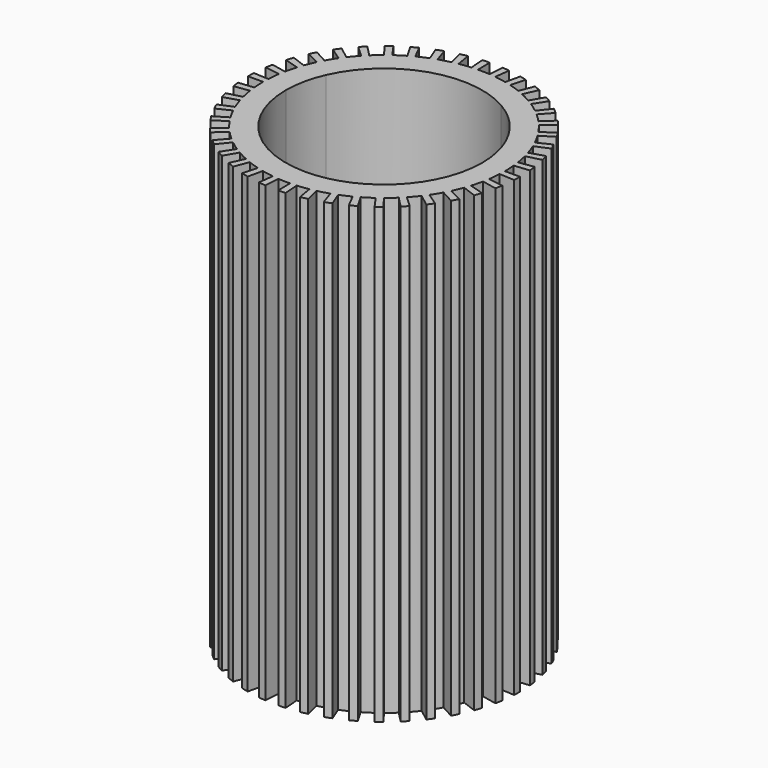
from build123d import *
from build123d import SkipClean  # not in build123d's __all__

# Parameters (mm, degrees)
F1_DEPTH = 1.5
F2_DEPTH = 30
F3_DEPTH = 10
F4_DEPTH = 10
F5_DEPTH = 1.5


with BuildPart() as f1:
    # F0 (on Top) → F1 (new body)
    with BuildSketch(Plane.XY):
        with BuildLine():
            ThreePointArc((-6.5, 0), (-4.3493489413, -4.8304413656), (0.6794350112, -6.4643923199))
            Line((0.6794350112, -6.4643923199), (0.3135853898, -2.9835656861))
            ThreePointArc((0.3135853898, -2.9835656861), (-2.0073918191, -2.2294344764), (-3, 0))
            Line((-3, 0), (-6.5, 0))
        make_face()
        with BuildLine():
            Line((-2.7406363729, 1.2202099292), (-5.9380454747, 2.64378818))
            ThreePointArc((-5.9380454747, 2.64378818), (-6.3579594048, 1.3514259903), (-6.5, 0))
            Line((-6.5, 0), (-3, 0))
            ThreePointArc((-3, 0), (-2.9344428022, 0.6237350725), (-2.7406363729, 1.2202099292))
        make_face()
        with BuildLine():
            Line((1.5, 2.5980762114), (3.25, 5.6291651246))
            ThreePointArc((3.25, 5.6291651246), (-2.0086104634, 6.1818673559), (-5.9380454747, 2.64378818))
            Line((-5.9380454747, 2.64378818), (-2.7406363729, 1.2202099292))
            ThreePointArc((-2.7406363729, 1.2202099292), (-0.9270509831, 2.8531695489), (1.5, 2.5980762114))
        make_face()
        with BuildLine():
            Line((2.4270509831, 1.7633557569), (5.2586104634, 3.8206041399))
            ThreePointArc((5.2586104634, 3.8206041399), (4.3493489413, 4.8304413656), (3.25, 5.6291651246))
            Line((3.25, 5.6291651246), (1.5, 2.5980762114))
            ThreePointArc((1.5, 2.5980762114), (2.0073918191, 2.2294344764), (2.4270509831, 1.7633557569))
        make_face()
        with BuildLine():
            ThreePointArc((3.25, -5.6291651246), (5.6291651246, -3.25), (6.5, 0))
            ThreePointArc((6.5, 0), (6.1818673559, 2.0086104634), (5.2586104634, 3.8206041399))
            Line((5.2586104634, 3.8206041399), (2.4270509831, 1.7633557569))
            ThreePointArc((2.4270509831, 1.7633557569), (2.8531695489, 0.9270509831), (3, 0))
            ThreePointArc((3, 0), (2.5980762114, -1.5), (1.5, -2.5980762114))
            Line((1.5, -2.5980762114), (3.25, -5.6291651246))
        make_face()
        with BuildLine():
            ThreePointArc((0.6794350112, -6.4643923199), (2.0086104634, -6.1818673559), (3.25, -5.6291651246))
            Line((3.25, -5.6291651246), (1.5, -2.5980762114))
            ThreePointArc((1.5, -2.5980762114), (0.9270509831, -2.8531695489), (0.3135853898, -2.9835656861))
            Line((0.3135853898, -2.9835656861), (0.6794350112, -6.4643923199))
        make_face()
    extrude(amount=F1_DEPTH)

    # F0 (on Top) → F2 (join)
    with BuildSketch(Plane.XY):
        with BuildLine():
            ThreePointArc((7.989036278, -0.4186876499), (7.9972585998, -0.2094155865), (8, 0))
            ThreePointArc((8, 0), (7.9905462891, 0.3888058656), (7.9622074997, 0.7766928166))
            ThreePointArc((7.9622074997, 0.7766928166), (7.9391476024, 0.9848529575), (7.9106466098, 1.1923381294))
            ThreePointArc((7.9106466098, 1.1923381294), (7.8433499818, 1.5753923522), (7.757516163, 1.9547232491))
            ThreePointArc((7.757516163, 1.9547232491), (7.7036891665, 2.1571215139), (7.6445824463, 2.3580413953))
            ThreePointArc((7.6445824463, 2.3580413953), (7.5209461966, 2.726787177), (7.3795347341, 3.0890883943))
            ThreePointArc((7.3795347341, 3.0890883943), (7.2961430447, 3.2812035401), (7.2077509432, 3.4710699129))
            ThreePointArc((7.2077509432, 3.4710699129), (7.0305369013, 3.8172700821), (6.8367066936, 4.1544484093))
            ThreePointArc((6.8367066936, 4.1544484093), (6.7256131437, 4.3319889013), (6.6099101945, 4.5065604645))
            ThreePointArc((6.6099101945, 4.5065604645), (6.3830770293, 4.8224814814), (6.1411579229, 5.1270049119))
            ThreePointArc((6.1411579229, 5.1270049119), (6.0048441589, 5.2860047888), (5.8644149746, 5.4413819022))
            ThreePointArc((5.8644149746, 5.4413819022), (5.5930297641, 5.7199666133), (5.3084258321, 5.9850325968))
            ThreePointArc((5.3084258321, 5.9850325968), (5.1499368782, 6.1219400643), (4.9879184149, 6.2546518597))
            ThreePointArc((4.9879184149, 6.2546518597), (4.6780434563, 6.4896771431), (4.3571122801, 6.7093645436))
            ThreePointArc((4.3571122801, 6.7093645436), (4.1799885177, 6.8211213148), (4, 6.9282032303))
            ThreePointArc((4, 6.9282032303), (3.6585573878, 7.1144190093), (3.3084680397, 7.2838203733))
            ThreePointArc((3.3084680397, 7.2838203733), (3.116666121, 7.3679299868), (2.9227281949, 7.4469899892))
            ThreePointArc((2.9227281949, 7.4469899892), (2.5573451929, 7.5802365111), (2.1859180904, 7.695567692))
            ThreePointArc((2.1859180904, 7.695567692), (1.9837225532, 7.750151278), (1.7801674717, 7.7994232975))
            ThreePointArc((1.7801674717, 7.7994232975), (1.3990061323, 7.8767240552), (1.0145383431, 7.935408745))
            ThreePointArc((1.0145383431, 7.935408745), (0.8064659016, 7.9592469964), (0.5978407487, 7.9776303774))
            ThreePointArc((0.5978407487, 7.9776303774), (0.2094155865, 7.9972585998), (-0.1795045144, 7.9979858795))
            ThreePointArc((-0.1795045144, 7.9979858795), (-0.3888058656, 7.9905462891), (-0.5978407487, 7.9776303774))
            ThreePointArc((-0.5978407487, 7.9776303774), (-0.9848529575, 7.9391476024), (-1.3695375376, 7.8819012258))
            ThreePointArc((-1.3695375376, 7.8819012258), (-1.5753923522, 7.8433499818), (-1.7801674717, 7.7994232975))
            ThreePointArc((-1.7801674717, 7.7994232975), (-2.1571215139, 7.7036891665), (-2.5289773553, 7.5897479231))
            ThreePointArc((-2.5289773553, 7.5897479231), (-2.726787177, 7.5209461966), (-2.9227281949, 7.4469899892))
            ThreePointArc((-2.9227281949, 7.4469899892), (-3.2812035401, 7.2961430447), (-3.6319239979, 7.1280521935))
            ThreePointArc((-3.6319239979, 7.1280521935), (-3.8172700821, 7.0305369013), (-4, 6.9282032303))
            ThreePointArc((-4, 6.9282032303), (-4.3319889013, 6.7256131437), (-4.65373946, 6.5071275567))
            ThreePointArc((-4.65373946, 6.5071275567), (-4.8224814814, 6.3830770293), (-4.9879184149, 6.2546518597))
            ThreePointArc((-4.9879184149, 6.2546518597), (-5.2860047888, 6.0048441589), (-5.5715980726, 5.7408444429))
            ThreePointArc((-5.5715980726, 5.7408444429), (-5.7199666133, 5.5930297641), (-5.8644149746, 5.4413819022))
            ThreePointArc((-5.8644149746, 5.4413819022), (-6.1219400643, 5.1499368782), (-6.3649963911, 4.8463203507))
            ThreePointArc((-6.3649963911, 4.8463203507), (-6.4896771431, 4.6780434563), (-6.6099101945, 4.5065604645))
            ThreePointArc((-6.6099101945, 4.5065604645), (-6.8211213148, 4.1799885177), (-7.016211208, 3.8435374702))
            ThreePointArc((-7.016211208, 3.8435374702), (-7.1144190093, 3.6585573878), (-7.2077509432, 3.4710699129))
            ThreePointArc((-7.2077509432, 3.4710699129), (-7.3679299868, 3.116666121), (-7.5106954604, 2.7548963139))
            ThreePointArc((-7.5106954604, 2.7548963139), (-7.5802365111, 2.5573451929), (-7.6445824463, 2.3580413953))
            ThreePointArc((-7.6445824463, 2.3580413953), (-7.750151278, 1.9837225532), (-7.8374031874, 1.6047153263))
            ThreePointArc((-7.8374031874, 1.6047153263), (-7.8767240552, 1.3990061323), (-7.9106466098, 1.1923381294))
            ThreePointArc((-7.9106466098, 1.1923381294), (-7.9592469964, 0.8064659016), (-7.989036278, 0.4186876499))
            ThreePointArc((-7.989036278, 0.4186876499), (-7.9972585998, 0.2094155865), (-8, 0))
            ThreePointArc((-8, 0), (-7.9905462891, -0.3888058656), (-7.9622074997, -0.7766928166))
            ThreePointArc((-7.9622074997, -0.7766928166), (-7.9391476024, -0.9848529575), (-7.9106466098, -1.1923381294))
            ThreePointArc((-7.9106466098, -1.1923381294), (-7.8433499818, -1.5753923522), (-7.757516163, -1.9547232491))
            ThreePointArc((-7.757516163, -1.9547232491), (-7.7036891665, -2.1571215139), (-7.6445824463, -2.3580413953))
            ThreePointArc((-7.6445824463, -2.3580413953), (-7.5209461966, -2.726787177), (-7.3795347341, -3.0890883943))
            ThreePointArc((-7.3795347341, -3.0890883943), (-7.2961430447, -3.2812035401), (-7.2077509432, -3.4710699129))
            ThreePointArc((-7.2077509432, -3.4710699129), (-7.0305369013, -3.8172700821), (-6.8367066936, -4.1544484093))
            ThreePointArc((-6.8367066936, -4.1544484093), (-6.7256131437, -4.3319889013), (-6.6099101945, -4.5065604645))
            ThreePointArc((-6.6099101945, -4.5065604645), (-6.3830770293, -4.8224814814), (-6.1411579229, -5.1270049119))
            ThreePointArc((-6.1411579229, -5.1270049119), (-6.0048441589, -5.2860047888), (-5.8644149746, -5.4413819022))
            ThreePointArc((-5.8644149746, -5.4413819022), (-5.5930297641, -5.7199666133), (-5.3084258321, -5.9850325968))
            ThreePointArc((-5.3084258321, -5.9850325968), (-5.1499368782, -6.1219400643), (-4.9879184149, -6.2546518597))
            ThreePointArc((-4.9879184149, -6.2546518597), (-4.6780434563, -6.4896771431), (-4.3571122801, -6.7093645436))
            ThreePointArc((-4.3571122801, -6.7093645436), (-4.1799885177, -6.8211213148), (-4, -6.9282032303))
            ThreePointArc((-4, -6.9282032303), (-3.6585573878, -7.1144190093), (-3.3084680397, -7.2838203733))
            ThreePointArc((-3.3084680397, -7.2838203733), (-3.116666121, -7.3679299868), (-2.9227281949, -7.4469899892))
            ThreePointArc((-2.9227281949, -7.4469899892), (-2.5573451929, -7.5802365111), (-2.1859180904, -7.695567692))
            ThreePointArc((-2.1859180904, -7.695567692), (-1.9837225532, -7.750151278), (-1.7801674717, -7.7994232975))
            ThreePointArc((-1.7801674717, -7.7994232975), (-1.3990061323, -7.8767240552), (-1.0145383431, -7.935408745))
            ThreePointArc((-1.0145383431, -7.935408745), (-0.8064659016, -7.9592469964), (-0.5978407487, -7.9776303774))
            ThreePointArc((-0.5978407487, -7.9776303774), (-0.2094155865, -7.9972585998), (0.1795045144, -7.9979858795))
            ThreePointArc((0.1795045144, -7.9979858795), (0.3888058656, -7.9905462891), (0.5978407487, -7.9776303774))
            ThreePointArc((0.5978407487, -7.9776303774), (0.9848529575, -7.9391476024), (1.3695375376, -7.8819012258))
            ThreePointArc((1.3695375376, -7.8819012258), (1.5753923522, -7.8433499818), (1.7801674717, -7.7994232975))
            ThreePointArc((1.7801674717, -7.7994232975), (2.1571215139, -7.7036891665), (2.5289773553, -7.5897479231))
            ThreePointArc((2.5289773553, -7.5897479231), (2.726787177, -7.5209461966), (2.9227281949, -7.4469899892))
            ThreePointArc((2.9227281949, -7.4469899892), (3.2812035401, -7.2961430447), (3.6319239979, -7.1280521935))
            ThreePointArc((3.6319239979, -7.1280521935), (3.8172700821, -7.0305369013), (4, -6.9282032303))
            ThreePointArc((4, -6.9282032303), (4.3319889013, -6.7256131437), (4.65373946, -6.5071275567))
            ThreePointArc((4.65373946, -6.5071275567), (4.8224814814, -6.3830770293), (4.9879184149, -6.2546518597))
            ThreePointArc((4.9879184149, -6.2546518597), (5.2860047888, -6.0048441589), (5.5715980726, -5.7408444429))
            ThreePointArc((5.5715980726, -5.7408444429), (5.7199666133, -5.5930297641), (5.8644149746, -5.4413819022))
            ThreePointArc((5.8644149746, -5.4413819022), (6.1219400643, -5.1499368782), (6.3649963911, -4.8463203507))
            ThreePointArc((6.3649963911, -4.8463203507), (6.4896771431, -4.6780434563), (6.6099101945, -4.5065604645))
            ThreePointArc((6.6099101945, -4.5065604645), (6.8211213148, -4.1799885177), (7.016211208, -3.8435374702))
            ThreePointArc((7.016211208, -3.8435374702), (7.1144190093, -3.6585573878), (7.2077509432, -3.4710699129))
            ThreePointArc((7.2077509432, -3.4710699129), (7.3679299868, -3.116666121), (7.5106954604, -2.7548963139))
            ThreePointArc((7.5106954604, -2.7548963139), (7.5802365111, -2.5573451929), (7.6445824463, -2.3580413953))
            ThreePointArc((7.6445824463, -2.3580413953), (7.750151278, -1.9837225532), (7.8374031874, -1.6047153263))
            ThreePointArc((7.8374031874, -1.6047153263), (7.8767240552, -1.3990061323), (7.9106466098, -1.1923381294))
            ThreePointArc((7.9106466098, -1.1923381294), (7.9592469964, -0.8064659016), (7.989036278, -0.4186876499))
        make_face()
        with BuildLine():
            ThreePointArc((5.2586104634, 3.8206041399), (6.1818673559, 2.0086104634), (6.5, 0))
            ThreePointArc((6.5, 0), (5.6291651246, -3.25), (3.25, -5.6291651246))
            ThreePointArc((3.25, -5.6291651246), (2.0086104634, -6.1818673559), (0.6794350112, -6.4643923199))
            ThreePointArc((0.6794350112, -6.4643923199), (-4.3493489413, -4.8304413656), (-6.5, 0))
            ThreePointArc((-6.5, 0), (-6.3579594048, 1.3514259903), (-5.9380454747, 2.64378818))
            ThreePointArc((-5.9380454747, 2.64378818), (-2.0086104634, 6.1818673559), (3.25, 5.6291651246))
            ThreePointArc((3.25, 5.6291651246), (4.3493489413, 4.8304413656), (5.2586104634, 3.8206041399))
        make_face(mode=Mode.SUBTRACT)
        with BuildLine():
            ThreePointArc((-6.6099101945, 4.5065604645), (-6.4896771431, 4.6780434563), (-6.3649963911, 4.8463203507))
            Line((-6.3649963911, 4.8463203507), (-7.1606209399, 5.4521103946))
            ThreePointArc((-7.1606209399, 5.4521103946), (-7.3008867859, 5.2627988883), (-7.4361489688, 5.0698805226))
            Line((-7.4361489688, 5.0698805226), (-6.6099101945, 4.5065604645))
        make_face()
        with BuildLine():
            ThreePointArc((-5.8644149746, 5.4413819022), (-5.7199666133, 5.5930297641), (-5.5715980726, 5.7408444429))
            Line((-5.5715980726, 5.7408444429), (-6.2680478317, 6.4584499982))
            ThreePointArc((-6.2680478317, 6.4584499982), (-6.43496244, 6.2921584847), (-6.5974668465, 6.1215546399))
            Line((-6.5974668465, 6.1215546399), (-5.8644149746, 5.4413819022))
        make_face()
        with BuildLine():
            ThreePointArc((-4.9879184149, 6.2546518597), (-4.8224814814, 6.3830770293), (-4.65373946, 6.5071275567))
            Line((-4.65373946, 6.5071275567), (-5.2354568925, 7.3205185012))
            ThreePointArc((-5.2354568925, 7.3205185012), (-5.4252916666, 7.1809616579), (-5.6114082167, 7.0364833422))
            Line((-5.6114082167, 7.0364833422), (-4.9879184149, 6.2546518597))
        make_face()
        with BuildLine():
            ThreePointArc((-4, 6.9282032303), (-3.8172700821, 7.0305369013), (-3.6319239979, 7.1280521935))
            Line((-3.6319239979, 7.1280521935), (-4.0859144977, 8.0190587177))
            ThreePointArc((-4.0859144977, 8.0190587177), (-4.2944288423, 7.909354014), (-4.5, 7.7942286341))
            Line((-4.5, 7.7942286341), (-4, 6.9282032303))
        make_face()
        with BuildLine():
            ThreePointArc((-2.9227281949, 7.4469899892), (-2.726787177, 7.5209461966), (-2.5289773553, 7.5897479231))
            Line((-2.5289773553, 7.5897479231), (-2.8450995247, 8.5384664135))
            ThreePointArc((-2.8450995247, 8.5384664135), (-3.0676355741, 8.4610644711), (-3.2880692193, 8.3778637378))
            Line((-3.2880692193, 8.3778637378), (-2.9227281949, 7.4469899892))
        make_face()
        with BuildLine():
            ThreePointArc((-1.7801674717, 7.7994232975), (-1.5753923522, 7.8433499818), (-1.3695375376, 7.8819012258))
            Line((-1.3695375376, 7.8819012258), (-1.5407297298, 8.867138879))
            ThreePointArc((-1.5407297298, 8.867138879), (-1.7723163963, 8.8237687295), (-2.0026884056, 8.7743512096))
            Line((-2.0026884056, 8.7743512096), (-1.7801674717, 7.7994232975))
        make_face()
        with BuildLine():
            ThreePointArc((-0.5978407487, 7.9776303774), (-0.3888058656, 7.9905462891), (-0.1795045144, 7.9979858795))
            Line((-0.1795045144, 7.9979858795), (-0.2019425787, 8.9977341145))
            ThreePointArc((-0.2019425787, 8.9977341145), (-0.4374065988, 8.9893645753), (-0.6725708423, 8.9748341746))
            Line((-0.6725708423, 8.9748341746), (-0.5978407487, 7.9776303774))
        make_face()
        with BuildLine():
            ThreePointArc((0.5978407487, 7.9776303774), (0.8064659016, 7.9592469964), (1.0145383431, 7.935408745))
            Line((1.0145383431, 7.935408745), (1.141355636, 8.9273348381))
            ThreePointArc((1.141355636, 8.9273348381), (0.9072741393, 8.9541528709), (0.6725708423, 8.9748341746))
            Line((0.6725708423, 8.9748341746), (0.5978407487, 7.9776303774))
        make_face()
        with BuildLine():
            ThreePointArc((1.7801674717, 7.7994232975), (1.9837225532, 7.750151278), (2.1859180904, 7.695567692))
            Line((2.1859180904, 7.695567692), (2.4591578517, 8.6575136535))
            ThreePointArc((2.4591578517, 8.6575136535), (2.2316878724, 8.7189201878), (2.0026884056, 8.7743512096))
            Line((2.0026884056, 8.7743512096), (1.7801674717, 7.7994232975))
        make_face()
        with BuildLine():
            ThreePointArc((2.9227281949, 7.4469899892), (3.116666121, 7.3679299868), (3.3084680397, 7.2838203733))
            Line((3.3084680397, 7.2838203733), (3.7220265447, 8.1942979199))
            ThreePointArc((3.7220265447, 8.1942979199), (3.5062493861, 8.2889212352), (3.2880692193, 8.3778637378))
            Line((3.2880692193, 8.3778637378), (2.9227281949, 7.4469899892))
        make_face()
        with BuildLine():
            ThreePointArc((4, 6.9282032303), (4.1799885177, 6.8211213148), (4.3571122801, 6.7093645436))
            Line((4.3571122801, 6.7093645436), (4.9017513151, 7.5480351115))
            ThreePointArc((4.9017513151, 7.5480351115), (4.7024870824, 7.6737614792), (4.5, 7.7942286341))
            Line((4.5, 7.7942286341), (4, 6.9282032303))
        make_face()
        with BuildLine():
            ThreePointArc((4.9879184149, 6.2546518597), (5.1499368782, 6.1219400643), (5.3084258321, 5.9850325968))
            Line((5.3084258321, 5.9850325968), (5.9719790611, 6.7331616714))
            ThreePointArc((5.9719790611, 6.7331616714), (5.793678988, 6.8871825723), (5.6114082167, 7.0364833422))
            Line((5.6114082167, 7.0364833422), (4.9879184149, 6.2546518597))
        make_face()
        with BuildLine():
            ThreePointArc((5.8644149746, 5.4413819022), (6.0048441589, 5.2860047888), (6.1411579229, 5.1270049119))
            Line((6.1411579229, 5.1270049119), (6.9088026632, 5.7678805259))
            ThreePointArc((6.9088026632, 5.7678805259), (6.7554496787, 5.9467553874), (6.5974668465, 6.1215546399))
            Line((6.5974668465, 6.1215546399), (5.8644149746, 5.4413819022))
        make_face()
        with BuildLine():
            ThreePointArc((6.6099101945, 4.5065604645), (6.7256131437, 4.3319889013), (6.8367066936, 4.1544484093))
            Line((6.8367066936, 4.1544484093), (7.6912950303, 4.6737544605))
            ThreePointArc((7.6912950303, 4.6737544605), (7.5663147867, 4.873487514), (7.4361489688, 5.0698805226))
            Line((7.4361489688, 5.0698805226), (6.6099101945, 4.5065604645))
        make_face()
        with BuildLine():
            ThreePointArc((7.2077509432, 3.4710699129), (7.2961430447, 3.2812035401), (7.3795347341, 3.0890883943))
            Line((7.3795347341, 3.0890883943), (8.3019765759, 3.4752244436))
            ThreePointArc((8.3019765759, 3.4752244436), (8.2081609253, 3.6913539826), (8.1087198111, 3.9049536521))
            Line((8.1087198111, 3.9049536521), (7.2077509432, 3.4710699129))
        make_face()
        with BuildLine():
            ThreePointArc((7.6445824463, 2.3580413953), (7.7036891665, 2.1571215139), (7.757516163, 1.9547232491))
            Line((7.757516163, 1.9547232491), (8.7272056834, 2.1990636552))
            ThreePointArc((8.7272056834, 2.1990636552), (8.6666503123, 2.4267617031), (8.6001552521, 2.6527965697))
            Line((8.6001552521, 2.6527965697), (7.6445824463, 2.3580413953))
        make_face()
        with BuildLine():
            ThreePointArc((7.9106466098, 1.1923381294), (7.9391476024, 0.9848529575), (7.9622074997, 0.7766928166))
            Line((7.9622074997, 0.7766928166), (8.9574834372, 0.8737794187))
            ThreePointArc((8.9574834372, 0.8737794187), (8.9315410527, 1.1079595772), (8.899477436, 1.3413803956))
            Line((8.899477436, 1.3413803956), (7.9106466098, 1.1923381294))
        make_face()
        with BuildLine():
            Line((9, 0), (8, 0))
            ThreePointArc((8, 0), (7.9972585998, -0.2094155865), (7.989036278, -0.4186876499))
            Line((7.989036278, -0.4186876499), (8.9876658128, -0.4710236062))
            ThreePointArc((8.9876658128, -0.4710236062), (8.9969159248, -0.2355925348), (9, 0))
        make_face()
        with BuildLine():
            Line((8.899477436, -1.3413803956), (7.9106466098, -1.1923381294))
            ThreePointArc((7.9106466098, -1.1923381294), (7.8767240552, -1.3990061323), (7.8374031874, -1.6047153263))
            Line((7.8374031874, -1.6047153263), (8.8170785858, -1.805304742))
            ThreePointArc((8.8170785858, -1.805304742), (8.8613145621, -1.5738818988), (8.899477436, -1.3413803956))
        make_face()
        with BuildLine():
            Line((8.6001552521, -2.6527965697), (7.6445824463, -2.3580413953))
            ThreePointArc((7.6445824463, -2.3580413953), (7.5802365111, -2.5573451929), (7.5106954604, -2.7548963139))
            Line((7.5106954604, -2.7548963139), (8.449532393, -3.0992583532))
            ThreePointArc((8.449532393, -3.0992583532), (8.527766075, -2.877013342), (8.6001552521, -2.6527965697))
        make_face()
        with BuildLine():
            Line((8.1087198111, -3.9049536521), (7.2077509432, -3.4710699129))
            ThreePointArc((7.2077509432, -3.4710699129), (7.1144190093, -3.6585573878), (7.016211208, -3.8435374702))
            Line((7.016211208, -3.8435374702), (7.893237609, -4.323979654))
            ThreePointArc((7.893237609, -4.323979654), (8.0037213855, -4.1158770613), (8.1087198111, -3.9049536521))
        make_face()
        with BuildLine():
            Line((7.4361489688, -5.0698805226), (6.6099101945, -4.5065604645))
            ThreePointArc((6.6099101945, -4.5065604645), (6.4896771431, -4.6780434563), (6.3649963911, -4.8463203507))
            Line((6.3649963911, -4.8463203507), (7.1606209399, -5.4521103946))
            ThreePointArc((7.1606209399, -5.4521103946), (7.3008867859, -5.2627988883), (7.4361489688, -5.0698805226))
        make_face()
        with BuildLine():
            Line((6.5974668465, -6.1215546399), (5.8644149746, -5.4413819022))
            ThreePointArc((5.8644149746, -5.4413819022), (5.7199666133, -5.5930297641), (5.5715980726, -5.7408444429))
            Line((5.5715980726, -5.7408444429), (6.2680478317, -6.4584499982))
            ThreePointArc((6.2680478317, -6.4584499982), (6.43496244, -6.2921584847), (6.5974668465, -6.1215546399))
        make_face()
        with BuildLine():
            Line((5.6114082167, -7.0364833422), (4.9879184149, -6.2546518597))
            ThreePointArc((4.9879184149, -6.2546518597), (4.8224814814, -6.3830770293), (4.65373946, -6.5071275567))
            Line((4.65373946, -6.5071275567), (5.2354568925, -7.3205185012))
            ThreePointArc((5.2354568925, -7.3205185012), (5.4252916666, -7.1809616579), (5.6114082167, -7.0364833422))
        make_face()
        with BuildLine():
            Line((4.5, -7.7942286341), (4, -6.9282032303))
            ThreePointArc((4, -6.9282032303), (3.8172700821, -7.0305369013), (3.6319239979, -7.1280521935))
            Line((3.6319239979, -7.1280521935), (4.0859144977, -8.0190587177))
            ThreePointArc((4.0859144977, -8.0190587177), (4.2944288423, -7.909354014), (4.5, -7.7942286341))
        make_face()
        with BuildLine():
            Line((3.2880692193, -8.3778637378), (2.9227281949, -7.4469899892))
            ThreePointArc((2.9227281949, -7.4469899892), (2.726787177, -7.5209461966), (2.5289773553, -7.5897479231))
            Line((2.5289773553, -7.5897479231), (2.8450995247, -8.5384664135))
            ThreePointArc((2.8450995247, -8.5384664135), (3.0676355741, -8.4610644711), (3.2880692193, -8.3778637378))
        make_face()
        with BuildLine():
            Line((2.0026884056, -8.7743512096), (1.7801674717, -7.7994232975))
            ThreePointArc((1.7801674717, -7.7994232975), (1.5753923522, -7.8433499818), (1.3695375376, -7.8819012258))
            Line((1.3695375376, -7.8819012258), (1.5407297298, -8.867138879))
            ThreePointArc((1.5407297298, -8.867138879), (1.7723163963, -8.8237687295), (2.0026884056, -8.7743512096))
        make_face()
        with BuildLine():
            Line((0.6725708423, -8.9748341746), (0.5978407487, -7.9776303774))
            ThreePointArc((0.5978407487, -7.9776303774), (0.3888058656, -7.9905462891), (0.1795045144, -7.9979858795))
            Line((0.1795045144, -7.9979858795), (0.2019425787, -8.9977341145))
            ThreePointArc((0.2019425787, -8.9977341145), (0.4374065988, -8.9893645753), (0.6725708423, -8.9748341746))
        make_face()
        with BuildLine():
            Line((-0.6725708423, -8.9748341746), (-0.5978407487, -7.9776303774))
            ThreePointArc((-0.5978407487, -7.9776303774), (-0.8064659016, -7.9592469964), (-1.0145383431, -7.935408745))
            Line((-1.0145383431, -7.935408745), (-1.141355636, -8.9273348381))
            ThreePointArc((-1.141355636, -8.9273348381), (-0.9072741393, -8.9541528709), (-0.6725708423, -8.9748341746))
        make_face()
        with BuildLine():
            Line((-2.0026884056, -8.7743512096), (-1.7801674717, -7.7994232975))
            ThreePointArc((-1.7801674717, -7.7994232975), (-1.9837225532, -7.750151278), (-2.1859180904, -7.695567692))
            Line((-2.1859180904, -7.695567692), (-2.4591578517, -8.6575136535))
            ThreePointArc((-2.4591578517, -8.6575136535), (-2.2316878724, -8.7189201878), (-2.0026884056, -8.7743512096))
        make_face()
        with BuildLine():
            Line((-3.2880692193, -8.3778637378), (-2.9227281949, -7.4469899892))
            ThreePointArc((-2.9227281949, -7.4469899892), (-3.116666121, -7.3679299868), (-3.3084680397, -7.2838203733))
            Line((-3.3084680397, -7.2838203733), (-3.7220265447, -8.1942979199))
            ThreePointArc((-3.7220265447, -8.1942979199), (-3.5062493861, -8.2889212352), (-3.2880692193, -8.3778637378))
        make_face()
        with BuildLine():
            Line((-4.5, -7.7942286341), (-4, -6.9282032303))
            ThreePointArc((-4, -6.9282032303), (-4.1799885177, -6.8211213148), (-4.3571122801, -6.7093645436))
            Line((-4.3571122801, -6.7093645436), (-4.9017513151, -7.5480351115))
            ThreePointArc((-4.9017513151, -7.5480351115), (-4.7024870824, -7.6737614792), (-4.5, -7.7942286341))
        make_face()
        with BuildLine():
            Line((-5.6114082167, -7.0364833422), (-4.9879184149, -6.2546518597))
            ThreePointArc((-4.9879184149, -6.2546518597), (-5.1499368782, -6.1219400643), (-5.3084258321, -5.9850325968))
            Line((-5.3084258321, -5.9850325968), (-5.9719790611, -6.7331616714))
            ThreePointArc((-5.9719790611, -6.7331616714), (-5.793678988, -6.8871825723), (-5.6114082167, -7.0364833422))
        make_face()
        with BuildLine():
            Line((-6.5974668465, -6.1215546399), (-5.8644149746, -5.4413819022))
            ThreePointArc((-5.8644149746, -5.4413819022), (-6.0048441589, -5.2860047888), (-6.1411579229, -5.1270049119))
            Line((-6.1411579229, -5.1270049119), (-6.9088026632, -5.7678805259))
            ThreePointArc((-6.9088026632, -5.7678805259), (-6.7554496787, -5.9467553874), (-6.5974668465, -6.1215546399))
        make_face()
        with BuildLine():
            Line((-7.4361489688, -5.0698805226), (-6.6099101945, -4.5065604645))
            ThreePointArc((-6.6099101945, -4.5065604645), (-6.7256131437, -4.3319889013), (-6.8367066936, -4.1544484093))
            Line((-6.8367066936, -4.1544484093), (-7.6912950303, -4.6737544605))
            ThreePointArc((-7.6912950303, -4.6737544605), (-7.5663147867, -4.873487514), (-7.4361489688, -5.0698805226))
        make_face()
        with BuildLine():
            Line((-8.1087198111, -3.9049536521), (-7.2077509432, -3.4710699129))
            ThreePointArc((-7.2077509432, -3.4710699129), (-7.2961430447, -3.2812035401), (-7.3795347341, -3.0890883943))
            Line((-7.3795347341, -3.0890883943), (-8.3019765759, -3.4752244436))
            ThreePointArc((-8.3019765759, -3.4752244436), (-8.2081609253, -3.6913539826), (-8.1087198111, -3.9049536521))
        make_face()
        with BuildLine():
            Line((-8.6001552521, -2.6527965697), (-7.6445824463, -2.3580413953))
            ThreePointArc((-7.6445824463, -2.3580413953), (-7.7036891665, -2.1571215139), (-7.757516163, -1.9547232491))
            Line((-7.757516163, -1.9547232491), (-8.7272056834, -2.1990636552))
            ThreePointArc((-8.7272056834, -2.1990636552), (-8.6666503123, -2.4267617031), (-8.6001552521, -2.6527965697))
        make_face()
        with BuildLine():
            Line((-8.899477436, -1.3413803956), (-7.9106466098, -1.1923381294))
            ThreePointArc((-7.9106466098, -1.1923381294), (-7.9391476024, -0.9848529575), (-7.9622074997, -0.7766928166))
            Line((-7.9622074997, -0.7766928166), (-8.9574834372, -0.8737794187))
            ThreePointArc((-8.9574834372, -0.8737794187), (-8.9315410527, -1.1079595772), (-8.899477436, -1.3413803956))
        make_face()
        with BuildLine():
            ThreePointArc((-8, 0), (-7.9972585998, 0.2094155865), (-7.989036278, 0.4186876499))
            Line((-7.989036278, 0.4186876499), (-8.9876658128, 0.4710236062))
            ThreePointArc((-8.9876658128, 0.4710236062), (-8.9969159248, 0.2355925348), (-9, 0))
            Line((-9, 0), (-8, 0))
        make_face()
        with BuildLine():
            ThreePointArc((-7.9106466098, 1.1923381294), (-7.8767240552, 1.3990061323), (-7.8374031874, 1.6047153263))
            Line((-7.8374031874, 1.6047153263), (-8.8170785858, 1.805304742))
            ThreePointArc((-8.8170785858, 1.805304742), (-8.8613145621, 1.5738818988), (-8.899477436, 1.3413803956))
            Line((-8.899477436, 1.3413803956), (-7.9106466098, 1.1923381294))
        make_face()
        with BuildLine():
            ThreePointArc((-7.6445824463, 2.3580413953), (-7.5802365111, 2.5573451929), (-7.5106954604, 2.7548963139))
            Line((-7.5106954604, 2.7548963139), (-8.449532393, 3.0992583532))
            ThreePointArc((-8.449532393, 3.0992583532), (-8.527766075, 2.877013342), (-8.6001552521, 2.6527965697))
            Line((-8.6001552521, 2.6527965697), (-7.6445824463, 2.3580413953))
        make_face()
        with BuildLine():
            ThreePointArc((-7.2077509432, 3.4710699129), (-7.1144190093, 3.6585573878), (-7.016211208, 3.8435374702))
            Line((-7.016211208, 3.8435374702), (-7.893237609, 4.323979654))
            ThreePointArc((-7.893237609, 4.323979654), (-8.0037213855, 4.1158770613), (-8.1087198111, 3.9049536521))
            Line((-8.1087198111, 3.9049536521), (-7.2077509432, 3.4710699129))
        make_face()
    extrude(amount=F2_DEPTH)

    # F0 (on Top) → F3 (join)
    with BuildSketch(Plane.XY):
        with BuildLine():
            ThreePointArc((3, 0), (2.8531695489, 0.9270509831), (2.4270509831, 1.7633557569))
            ThreePointArc((2.4270509831, 1.7633557569), (2.0073918191, 2.2294344764), (1.5, 2.5980762114))
            ThreePointArc((1.5, 2.5980762114), (-0.9270509831, 2.8531695489), (-2.7406363729, 1.2202099292))
            ThreePointArc((-2.7406363729, 1.2202099292), (-2.9344428022, 0.6237350725), (-3, 0))
            ThreePointArc((-3, 0), (-2.0073918191, -2.2294344764), (0.3135853898, -2.9835656861))
            ThreePointArc((0.3135853898, -2.9835656861), (0.9270509831, -2.8531695489), (1.5, -2.5980762114))
            ThreePointArc((1.5, -2.5980762114), (2.5980762114, -1.5), (3, 0))
        make_face()
        with BuildLine():
            ThreePointArc((1.1180339887, 1), (0, -1.5), (-1.1180339887, 1))
            Line((-1.1180339887, 1), (1.1180339887, 1))
        make_face(mode=Mode.SUBTRACT)
    extrude(amount=F3_DEPTH)

    # F0 (on Top) → F4 (join)
    with BuildSketch(Plane.XY):
        with BuildLine():
            Line((-2.7406363729, 1.2202099292), (-5.9380454747, 2.64378818))
            ThreePointArc((-5.9380454747, 2.64378818), (-6.3579594048, 1.3514259903), (-6.5, 0))
            Line((-6.5, 0), (-3, 0))
            ThreePointArc((-3, 0), (-2.9344428022, 0.6237350725), (-2.7406363729, 1.2202099292))
        make_face()
        with BuildLine():
            Line((2.4270509831, 1.7633557569), (5.2586104634, 3.8206041399))
            ThreePointArc((5.2586104634, 3.8206041399), (4.3493489413, 4.8304413656), (3.25, 5.6291651246))
            Line((3.25, 5.6291651246), (1.5, 2.5980762114))
            ThreePointArc((1.5, 2.5980762114), (2.0073918191, 2.2294344764), (2.4270509831, 1.7633557569))
        make_face()
        with BuildLine():
            ThreePointArc((0.6794350112, -6.4643923199), (2.0086104634, -6.1818673559), (3.25, -5.6291651246))
            Line((3.25, -5.6291651246), (1.5, -2.5980762114))
            ThreePointArc((1.5, -2.5980762114), (0.9270509831, -2.8531695489), (0.3135853898, -2.9835656861))
            Line((0.3135853898, -2.9835656861), (0.6794350112, -6.4643923199))
        make_face()
    extrude(amount=F4_DEPTH)

    # F0 (on Top) → F5 (cut)
    with BuildSketch(Plane.XY):
        with BuildLine():
            ThreePointArc((3.25, -5.6291651246), (5.6291651246, -3.25), (6.5, 0))
            ThreePointArc((6.5, 0), (6.1818673559, 2.0086104634), (5.2586104634, 3.8206041399))
            Line((5.2586104634, 3.8206041399), (2.4270509831, 1.7633557569))
            ThreePointArc((2.4270509831, 1.7633557569), (2.8531695489, 0.9270509831), (3, 0))
            ThreePointArc((3, 0), (2.5980762114, -1.5), (1.5, -2.5980762114))
            Line((1.5, -2.5980762114), (3.25, -5.6291651246))
        make_face()
        with BuildLine():
            ThreePointArc((-6.5, 0), (-4.3493489413, -4.8304413656), (0.6794350112, -6.4643923199))
            Line((0.6794350112, -6.4643923199), (0.3135853898, -2.9835656861))
            ThreePointArc((0.3135853898, -2.9835656861), (-2.0073918191, -2.2294344764), (-3, 0))
            Line((-3, 0), (-6.5, 0))
        make_face()
        with BuildLine():
            Line((1.5, 2.5980762114), (3.25, 5.6291651246))
            ThreePointArc((3.25, 5.6291651246), (-2.0086104634, 6.1818673559), (-5.9380454747, 2.64378818))
            Line((-5.9380454747, 2.64378818), (-2.7406363729, 1.2202099292))
            ThreePointArc((-2.7406363729, 1.2202099292), (-0.9270509831, 2.8531695489), (1.5, 2.5980762114))
        make_face()
    with SkipClean():  # cleaning this boolean's faces spoils the solid; the shape is the same uncleaned
        extrude(amount=F5_DEPTH, mode=Mode.SUBTRACT)


solid = f1.part
